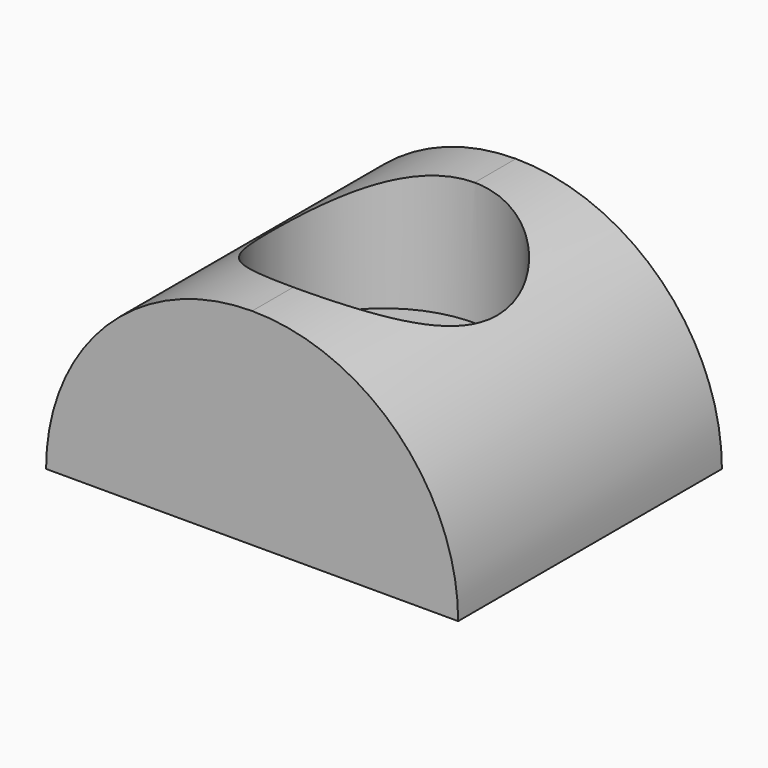
from build123d import *

# Parameters (mm, degrees)
F0_W     = 10
F0_H     = 8
F1_DEPTH = 5
F2_R     = 4.99999
F3_R     = 1.5
F5_DEPTH = 5
F6_R     = 2.75
F7_DEPTH = 3


# Not quite as in the source:
# - a fillet or chamfer is up to 0.001 mm smaller than in the source, because OpenCascade refuses the exact size


with BuildPart() as f1:
    # F0 (on Top) → F1 (new body)
    with BuildSketch(Plane.XY):
        with Locations((5, 4)):
            Rectangle(F0_W, F0_H)
    extrude(amount=F1_DEPTH)

    # F2 (radius 5 in the source; OpenCascade refuses exactly that, so slightly less here)
    f2_edges = [f1.edges().sort_by_distance(p)[0] for p in [
        (0, 4, 5),
        (10, 4, 5),
    ]]
    fillet(f2_edges, radius=F2_R)

    # F3 (on face) → F5 (cut)
    with BuildSketch(Plane(origin=(0, 0, 0), x_dir=(1, 0, 0), z_dir=(0, 0, -1))):
        with Locations((5, -4)):
            Circle(F3_R)
    extrude(amount=-F5_DEPTH, mode=Mode.SUBTRACT)

    # F6 (on offset) → F7 (cut)
    with BuildSketch(Plane.XY.offset(5)):
        with Locations((5, 4)):
            Circle(F6_R)
    extrude(amount=-F7_DEPTH, mode=Mode.SUBTRACT)


solid = f1.part
